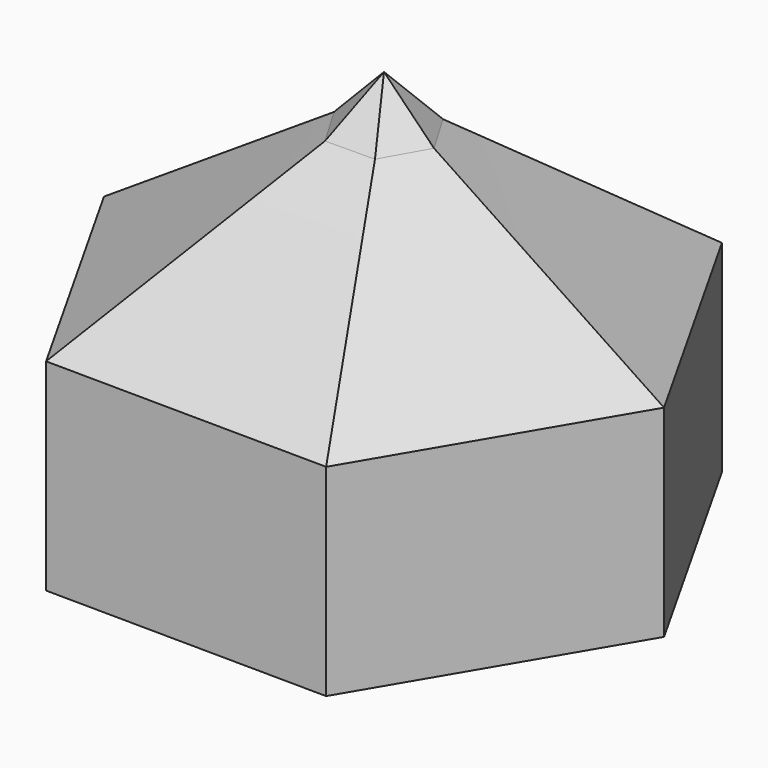
from build123d import *

# Parameters (mm, degrees)
F2_DEPTH = 50.8
F5_DEPTH = 50.8
F5_TAPER = 40


with BuildPart() as f2:
    # F1 (on Top) → F2 (new body)
    with BuildSketch(Plane.XY):
        Polygon((71.0278424351, -0.688096386), (36.109830168, 61.1678677318), (-34.9180122671, 61.8559641178), (-71.0278424351, 0.688096386), (-36.109830168, -61.1678677318), (34.9180122671, -61.8559641178), align=None)
    extrude(amount=-F2_DEPTH)

    # F3 (on offset) → F4 section 0
    with BuildSketch(Plane.XY.offset(38.1)):
        Polygon((6.3483007252, -10.7696512714), (12.5009419535, 0.1129640632), (6.1526412283, 10.8826153346), (-6.3483007252, 10.7696512714), (-12.5009419535, -0.1129640632), (-6.1526412283, -10.8826153346), align=None)
    # F2_face (on face) → F4 section 1
    with BuildSketch(Plane.XY):
        Polygon((71.0278424351, -0.688096386), (36.109830168, 61.1678677318), (-34.9180122671, 61.8559641178), (-71.0278424351, 0.688096386), (-36.109830168, -61.1678677318), (34.9180122671, -61.8559641178), align=None)
    loft()

    # F4_face (on face) → F5 (join)
    with BuildSketch(Plane.XY.offset(38.1)):
        Polygon((-6.1526412283, -10.8826153346), (6.3483007252, -10.7696512714), (12.5009419535, 0.1129640632), (6.1526412283, 10.8826153346), (-6.3483007252, 10.7696512714), (-12.5009419535, -0.1129640632), align=None)
    extrude(amount=F5_DEPTH, taper=F5_TAPER)


solid = f2.part
